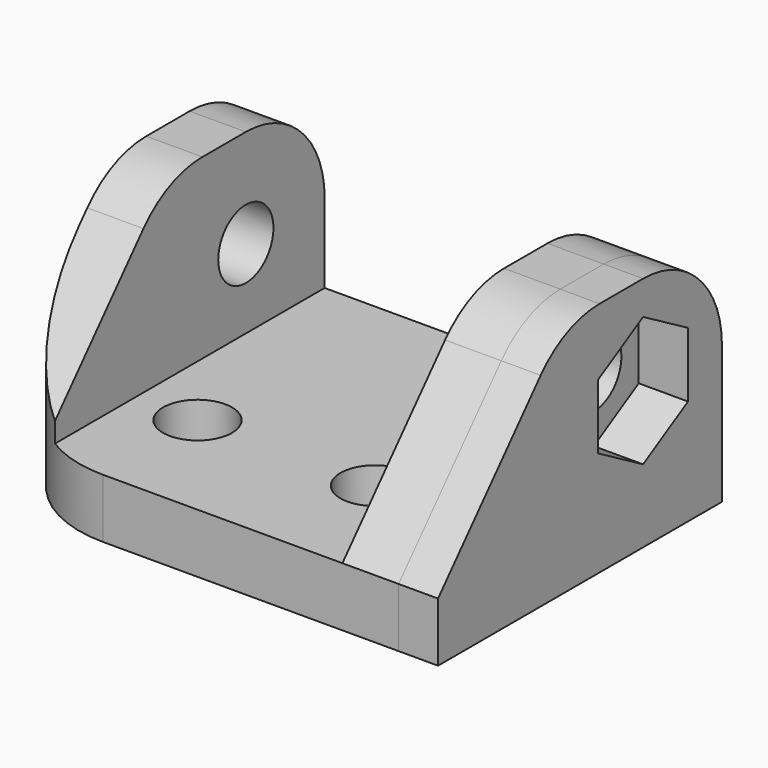
from build123d import *

# Parameters (mm, degrees)
F0_W      = 21
F0_H      = 18
F1_DEPTH  = 3
F2_W      = 2.85
F2_H      = 18
F3_DEPTH  = 9
F4_R      = 6
F5_R      = 1.75
F6_DEPTH  = 21.001
F7_R      = 5
F8_R      = 1.75
F9_DEPTH  = 3.001
F10_DEPTH = 2
F12_DEPTH = 2.5


with BuildPart() as f1:
    # F0 (on Top) → F1 (new body)
    with BuildSketch(Plane.XY):
        with Locations((10.5, 9)):
            Rectangle(F0_W, F0_H)
    extrude(amount=F1_DEPTH)

    # F2 (on face) → F3 (join)
    with BuildSketch(Plane.XY.offset(3)):
        with Locations((1.425, 9)):
            Rectangle(F2_W, F2_H)
        with Locations((19.575, 9)):
            Rectangle(F2_W, F2_H)
    extrude(amount=F3_DEPTH)

    # F4
    f4_edges = [f1.edges().sort_by_distance(p)[0] for p in [
        (0, 0, 6),
    ]]
    fillet(f4_edges, radius=F4_R)

    # F5 (on face) → F6 (cut, through all)
    with BuildSketch(Plane(origin=(0, 0, 0), x_dir=(0, -1, 0), z_dir=(-1, 0, 0))):
        with Locations((-13, 7)):
            Circle(F5_R)
        Polygon((0, 12), (-8, 12), (0, 3), align=None)
    extrude(amount=-F6_DEPTH, mode=Mode.SUBTRACT)

    # F7
    f7_edges = [f1.edges().sort_by_distance(p)[0] for p in [
        (1.425, 18, 12),
        (19.575, 18, 12),
        (1.425, 8, 12),
        (19.575, 8, 12),
    ]]
    fillet(f7_edges, radius=F7_R)

    # F8 (on face) → F9 (cut, through all)
    with BuildSketch(Plane.XY.offset(3)):
        with Locations((6, 6)):
            Circle(F8_R)
        with Locations((15, 6)):
            Circle(F8_R)
    extrude(amount=-F9_DEPTH, mode=Mode.SUBTRACT)

    # F10 (add): a face of the model
    f10_faces = [f1.faces().sort_by_distance(p)[0] for p in [
        (21, 9.8993100801, 5.1016484072),
    ]]
    extrude(f10_faces, amount=F10_DEPTH)

    # F11 (on face) → F12 (cut)
    with BuildSketch(Plane.YZ.offset(23)):
        Polygon((15.85, 5.3545517328), (15.85, 8.6454482672), (13, 10.2908965344), (10.15, 8.6454482672), (10.15, 5.3545517328), (13, 3.7091034656), align=None)
    extrude(amount=-F12_DEPTH, mode=Mode.SUBTRACT)


solid = f1.part
